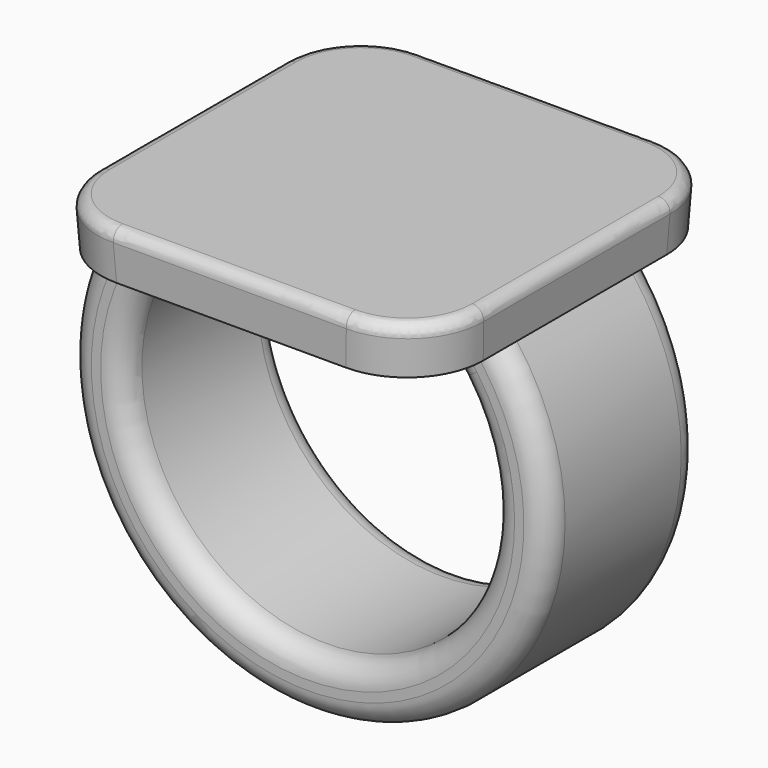
from build123d import *

# Parameters (mm, degrees)
F0_W          = 25.4
F0_H          = 25.4
F1_DEPTH      = 3.175
F1_TAPER      = -3
F3_W          = 5.08
F3_H          = 12.7
F6_DEPTH      = 6.35
F6_DEPTH_BACK = 6.35
F7_R          = 5.08
F8_R          = 1.524
F9_R          = 0.762


with BuildPart() as f1:
    # F0 (on Top) → F1 (new body)
    with BuildSketch(Plane.XY):
        Rectangle(F0_W, F0_H)
    extrude(amount=F1_DEPTH, taper=F1_TAPER)

    # F4: sweep along a path in F2
    with BuildLine(Plane.XZ) as f4_path:
        ThreePointArc((-10.16, 0), (0, -23.5582897328), (10.16, 0))
    # F3 (on face) → F4 (sweep)
    with BuildSketch(Plane(origin=(0, 0, 0), x_dir=(1, 0, 0), z_dir=(0, 0, -1))):
        with Locations((-10.16, 0)):
            Rectangle(F3_W, F3_H)
    sweep(path=f4_path.line)

    # F5 (on Front) → F6 (join, two sides)
    with BuildSketch(Plane.XZ) as f6_sk:
        with BuildLine():
            ThreePointArc((7.62, 0), (8.9072265211, -1.1822790439), (10.0130578512, -2.535746045))
            Line((10.0130578512, -2.535746045), (10.16, 0))
            Line((10.16, 0), (7.62, 0))
        make_face()
    extrude(amount=F6_DEPTH)
    extrude(f6_sk.sketch, amount=-F6_DEPTH_BACK)

    # F7
    f7_edges = [f1.edges().sort_by_distance(p)[0] for p in [
        (-12.783197, -12.783197, 1.5875),
        (12.783197, -12.783197, 1.5875),
        (12.783197, 12.783197, 1.5875),
        (-12.783197, 12.783197, 1.5875),
    ]]
    fillet(f7_edges, radius=F7_R)

    # F8
    f8_edges = [f1.edges().sort_by_distance(p)[0] for p in [
        (-1.743325, -6.35, -21.711017),
        (8.907227, -6.35, -1.182279),
        (-1.743325, 6.35, -21.711017),
        (8.907227, 6.35, -1.182279),
        (0, 6.35, -25.501344),
        (0, -6.35, -25.501344),
    ]]
    fillet(f8_edges, radius=F8_R)

    # F9
    f9_edges = [f1.edges().sort_by_distance(p)[0] for p in [
        (0, 12.866395, 3.175),
        (11.381378, 11.381378, 3.175),
        (-11.381378, 11.381378, 3.175),
        (12.866395, 0, 3.175),
        (-12.866395, 0, 3.175),
        (11.381378, -11.381378, 3.175),
        (-11.381378, -11.381378, 3.175),
        (0, -12.866395, 3.175),
    ]]
    fillet(f9_edges, radius=F9_R)


solid = f1.part
